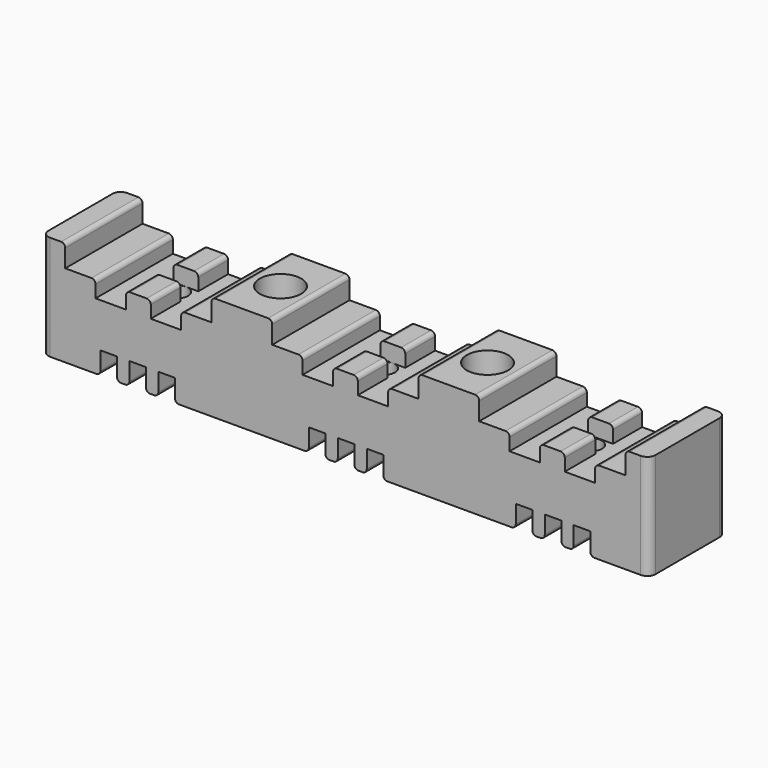
from build123d import *

# Parameters (mm, degrees)
F1_DEPTH         = 17.5
F4_D             = 8.8
F4_ON_F3_D       = 8.8
F7_D             = 15
F7_DEPTH         = 12
F7_TIP           = 4.5064546427
F8_D             = 15
F8_DEPTH         = 12
F8_TIP           = 4.5064546427
F11_D            = 15
F11_DEPTH        = 12
F11_TIP          = 4.5064546427
F12_D            = 15
F12_DEPTH        = 12
F12_TIP          = 4.5064546427
F13_W            = 9
F13_H            = 8
F13_W_2          = 10
F14_DEPTH        = 6
F16_D            = 8
F16_DEPTH        = 12
F16_TIP          = 2.4034424761
F17_W            = 9
F17_H            = 8
F18_DEPTH        = 6
F19_W            = 9
F19_H            = 8
F20_DEPTH        = 6
F23_D            = 8
F23_DEPTH        = 12
F23_TIP          = 2.4034424761
F23_ON_F21_D     = 8
F23_ON_F21_DEPTH = 12
F23_ON_F21_TIP   = 2.4034424761
F27_DEPTH        = 8
F31_D            = 15
F31_DEPTH        = 5
F31_TIP          = 4.5064546427
F31_ON_F29_D     = 15
F31_ON_F29_DEPTH = 5
F31_ON_F29_TIP   = 4.5064546427
F31_ON_F30_D     = 15
F31_ON_F30_DEPTH = 5
F31_ON_F30_TIP   = 4.5064546427
F32_R            = 3
F33_R            = 1.5


# Not quite as in the source:
# - a feature names something its author has since deleted; it is built from what else it names


with BuildPart() as f1:
    # F0 (on Front) → F1 (new body, symmetric)
    with BuildSketch(Plane.XZ):
        Polygon((0.5, 11), (0.5, 5), (-10.5, 5), (-10.5, 11), (-21.5, 11), (-21.5, 19), (-43.5, 19), (-43.5, 11), (-54.5, 11), (-54.5, 5), (-65.5, 5), (-65.5, 11), (-74.5, 11), (-74.5, 5), (-85.5, 5), (-85.5, 11), (-96.5, 11), (-96.5, 19), (-105, 19), (-105, -19), (-83.75, -19), (-83.75, -11), (-77.75, -11), (-77.75, -19), (-73.25, -19), (-73.25, -11), (-67.25, -11), (-67.25, -19), (-62.75, -19), (-62.75, -11), (-56.75, -11), (-56.75, -19), (-8.25, -19), (-8.25, -11), (-2.25, -11), (-2.25, -19), (2.25, -19), (2.25, -11), (8.25, -11), (8.25, -19), (12.75, -19), (12.75, -11), (18.75, -11), (18.75, -19), (66.75, -19), (66.75, -11), (72.75, -11), (72.75, -19), (77.25, -19), (77.25, -11), (83.25, -11), (83.25, -19), (87.75, -19), (87.75, -11), (93.75, -11), (93.75, -19), (115, -19), (115, 19), (106.5, 19), (106.5, 11), (95.5, 11), (95.5, 5), (84.5, 5), (84.5, 11), (75.5, 11), (75.5, 5), (64.5, 5), (64.5, 11), (53.5, 11), (53.5, 19), (31.5, 19), (31.5, 11), (20.5, 11), (20.5, 5), (9.5, 5), (9.5, 11), align=None)
    extrude(amount=F1_DEPTH, both=True)

    # F4 (through all)
    with Locations(Plane.XY.offset(19)):
        with Locations((-32.5, 0)):
            Hole(F4_D / 2)

    # F4 on F3 (through all)
    with Locations(Plane.XY.offset(19)):
        with Locations((42.5, 0)):
            Hole(F4_ON_F3_D / 2)

    # F7
    with Locations(Plane.XY.offset(19)):
        with Locations((-32.5, 0)):
            Hole(F7_D / 2, depth=F7_DEPTH)
            with Locations((0, 0, -(F7_DEPTH + F7_TIP / 2))):  # 118° drill point
                Cone(0, F7_D / 2, F7_TIP, mode=Mode.SUBTRACT)

    # F8
    with Locations(Plane.XY.offset(19)):
        with Locations((42.5, 0)):
            Hole(F8_D / 2, depth=F8_DEPTH)
            with Locations((0, 0, -(F8_DEPTH + F8_TIP / 2))):  # 118° drill point
                Cone(0, F8_D / 2, F8_TIP, mode=Mode.SUBTRACT)

    # F11
    with Locations(Plane(origin=(0, 0, -19), x_dir=(1, 0, 0), z_dir=(0, 0, -1))):
        with Locations((42.5, 0)):
            Hole(F11_D / 2, depth=F11_DEPTH)
            with Locations((0, 0, -(F11_DEPTH + F11_TIP / 2))):  # 118° drill point
                Cone(0, F11_D / 2, F11_TIP, mode=Mode.SUBTRACT)

    # F12
    with Locations(Plane(origin=(0, 0, -19), x_dir=(1, 0, 0), z_dir=(0, 0, -1))):
        with Locations((-32.5, 0)):
            Hole(F12_D / 2, depth=F12_DEPTH)
            with Locations((0, 0, -(F12_DEPTH + F12_TIP / 2))):  # 118° drill point
                Cone(0, F12_D / 2, F12_TIP, mode=Mode.SUBTRACT)

    # F13 (on face) → F14 (cut)
    with BuildSketch(Plane.XY.offset(11)):
        with Locations((5, 0)):
            Rectangle(F13_W, F13_H)
        with Locations((-4.5, 0)):
            Rectangle(F13_W_2, F13_H)
    extrude(amount=-F14_DEPTH, mode=Mode.SUBTRACT)

    # F16
    with Locations(Plane.XY.offset(5)):
        with Locations((5, 0)):
            Hole(F16_D / 2, depth=F16_DEPTH)
            with Locations((0, 0, -(F16_DEPTH + F16_TIP / 2))):  # 118° drill point
                Cone(0, F16_D / 2, F16_TIP, mode=Mode.SUBTRACT)

    # F17 (on face) → F18 (cut)
    with BuildSketch(Plane.XY.offset(11)):
        with Locations((80, 0.3464802131)):
            Rectangle(F17_W, F17_H)
    extrude(amount=-F18_DEPTH, mode=Mode.SUBTRACT)

    # F19 (on face) → F20 (cut)
    with BuildSketch(Plane.XY.offset(11)):
        with Locations((-70, 0)):
            Rectangle(F19_W, F19_H)
    extrude(amount=-F20_DEPTH, mode=Mode.SUBTRACT)

    # F23
    with Locations(Plane.XY.offset(5)):
        with Locations((-70, 0)):
            Hole(F23_D / 2, depth=F23_DEPTH)
            with Locations((0, 0, -(F23_DEPTH + F23_TIP / 2))):  # 118° drill point
                Cone(0, F23_D / 2, F23_TIP, mode=Mode.SUBTRACT)

    # F23 on F21 (one way)
    with BuildSketch(Plane.XY.offset(5)):
        with Locations((80, 0)):
            Circle(F23_ON_F21_D / 2)
    extrude(amount=-F23_ON_F21_DEPTH, mode=Mode.SUBTRACT)
    with Locations(Plane.XY.offset(5)):
        with Locations((80, 0)):
            with Locations((0, 0, -(F23_ON_F21_DEPTH + F23_ON_F21_TIP / 2))):  # 118° drill point
                Cone(0, F23_ON_F21_D / 2, F23_ON_F21_TIP, mode=Mode.SUBTRACT)

    # F24 (on face) + F25 (on face) + F26 (on face) → F27 (cut)
    with BuildSketch(Plane(origin=(0, 0, -19), x_dir=(1, 0, 0), z_dir=(0, 0, -1))):
        Polygon((-73.25, 0), (-73.25, 7.5), (-77.75, 7.5), (-77.75, -7.5), (-73.25, -7.5), align=None)
        Polygon((-62.75, -7.5), (-62.75, 7.5), (-73.25, 7.5), (-73.25, 0), (-73.25, -7.5), align=None)
    with BuildSketch(Plane(origin=(0, 0, -19), x_dir=(1, 0, 0), z_dir=(0, 0, -1))):
        Polygon((-2.25, -7.5), (2.25, -7.5), (2.25, 0), (2.25, 7.5), (-2.25, 7.5), align=None)
        Polygon((2.25, -7.5), (12.75, -7.5), (12.75, 7.5), (2.25, 7.5), (2.25, 0), align=None)
    with BuildSketch(Plane(origin=(0, 0, -19), x_dir=(1, 0, 0), z_dir=(0, 0, -1))):
        Polygon((77.25, 0), (77.25, 7.5), (72.75, 7.5), (72.75, -7.5), (77.25, -7.5), align=None)
        Polygon((87.75, -7.5), (87.75, 7.5), (77.25, 7.5), (77.25, 0), (77.25, -7.5), align=None)
    extrude(amount=-F27_DEPTH, mode=Mode.SUBTRACT)

    # F31
    with Locations(Plane(origin=(0, 0, -11), x_dir=(1, 0, 0), z_dir=(0, 0, -1))):
        with Locations((-70.25, 0)):
            Hole(F31_D / 2, depth=F31_DEPTH)
            with Locations((0, 0, -(F31_DEPTH + F31_TIP / 2))):  # 118° drill point
                Cone(0, F31_D / 2, F31_TIP, mode=Mode.SUBTRACT)

    # F31 on F29
    with Locations(Plane(origin=(0, 0, -11), x_dir=(1, 0, 0), z_dir=(0, 0, -1))):
        with Locations((5.25, 0)):
            Hole(F31_ON_F29_D / 2, depth=F31_ON_F29_DEPTH)
            with Locations((0, 0, -(F31_ON_F29_DEPTH + F31_ON_F29_TIP / 2))):  # 118° drill point
                Cone(0, F31_ON_F29_D / 2, F31_ON_F29_TIP, mode=Mode.SUBTRACT)

    # F31 on F30
    with Locations(Plane(origin=(0, 0, -11), x_dir=(1, 0, 0), z_dir=(0, 0, -1))):
        with Locations((80.25, 0)):
            Hole(F31_ON_F30_D / 2, depth=F31_ON_F30_DEPTH)
            with Locations((0, 0, -(F31_ON_F30_DEPTH + F31_ON_F30_TIP / 2))):  # 118° drill point
                Cone(0, F31_ON_F30_D / 2, F31_ON_F30_TIP, mode=Mode.SUBTRACT)

    # F32
    f32_edges = [f1.edges().sort_by_distance(p)[0] for p in [
        (-105, -17.5, 0),
        (-105, 17.5, 0),
        (115, -17.5, 0),
        (115, 17.5, 0),
    ]]
    fillet(f32_edges, radius=F32_R)

    # F33
    f33_edges = [f1.edges().sort_by_distance(p)[0] for p in [
        (93.75, 0, -19),
        (66.75, 0, -19),
        (18.75, 0, -19),
        (-8.25, 0, -19),
        (-56.75, 0, -19),
        (-83.75, 0, -19),
        (-77.75, 12.5, -19),
        (-73.25, 12.5, -19),
        (-67.25, 12.5, -19),
        (-62.75, 12.5, -19),
        (-62.75, -12.5, -19),
        (-67.25, -12.5, -19),
        (-73.25, -12.5, -19),
        (-77.75, -12.5, -19),
        (-2.25, 12.5, -19),
        (2.25, 12.5, -19),
        (8.25, 12.5, -19),
        (12.75, 12.5, -19),
        (8.25, -12.5, -19),
        (2.25, -12.5, -19),
        (-2.25, -12.5, -19),
        (72.75, -12.5, -19),
        (77.25, -12.5, -19),
        (83.25, -12.5, -19),
        (87.75, -12.5, -19),
        (87.75, 12.5, -19),
        (83.25, 12.5, -19),
        (77.25, 12.5, -19),
        (72.75, 12.5, -19),
        (12.75, -12.5, -19),
        (-21.5, 0, 19),
        (53.5, 0, 19),
        (31.5, 0, 19),
        (-43.5, 0, 19),
        (-65.5, 10.75, 11),
        (-65.5, -10.75, 11),
        (-74.5, -10.75, 11),
        (-74.5, 10.75, 11),
        (-85.5, 0, 11),
        (-96.5, 0, 19),
        (-10.5, 0, 11),
        (0.5, -10.75, 11),
        (0.5, 10.75, 11),
        (9.5, 10.75, 11),
        (9.5, -10.75, 11),
        (20.5, 0, 11),
        (64.5, 0, 11),
        (84.5, -10.57676, 11),
        (75.5, -10.57676, 11),
        (84.5, 10.92324, 11),
        (75.5, 10.92324, 11),
        (106.5, 0, 19),
        (95.5, 0, 11),
        (-54.5, 0, 11),
    ]]
    fillet(f33_edges, radius=F33_R)


solid = f1.part
